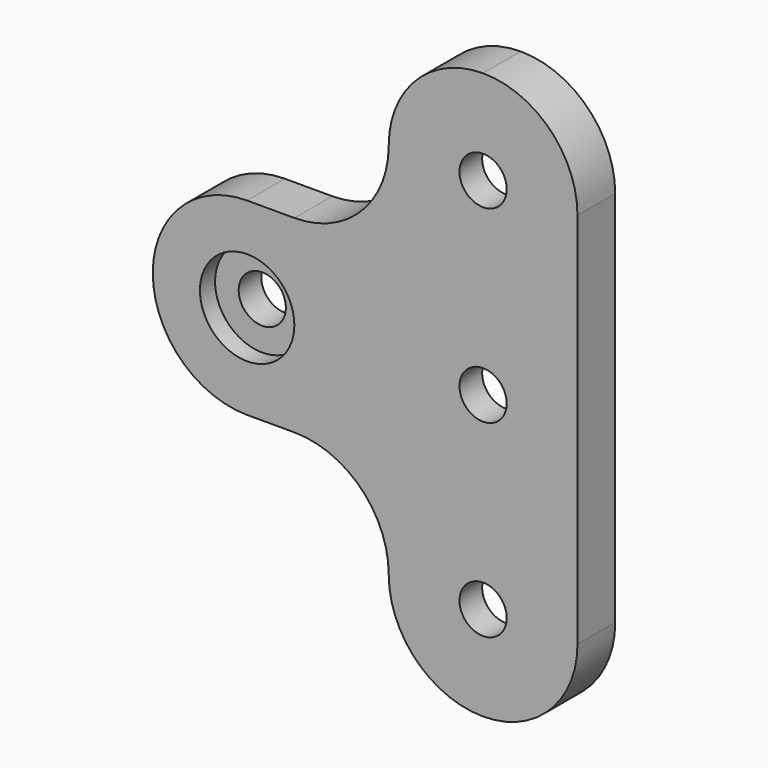
from build123d import *

# Parameters (mm, degrees)
F1_DEPTH       = 5
F2_D           = 5
F2_CBORE_D     = 10
F2_CBORE_DEPTH = 2
F3_R           = 9.99999
F5_D           = 5
F5_CBORE_D     = 10
F5_CBORE_DEPTH = 2


# Not quite as in the source:
# - a fillet or chamfer is up to 0.001 mm smaller than in the source, because OpenCascade refuses the exact size


with BuildPart() as f1:
    # F0 (on Front) → F1 (new body)
    with BuildSketch(Plane.XZ):
        Polygon((15, 10), (-10, 10), (-10, -10), (15, -10), (15, -30), (35, -30), (35, -10), (35, 10), (35, 30), (15, 30), align=None)
    extrude(amount=F1_DEPTH)

    # F2 (through all)
    with Locations(Plane(origin=(0, 0, 0), x_dir=(1, 0, 0), z_dir=(0, 1, 0))):
        with Locations((25, -20), (25, 20), (25, 0)):
            CounterBoreHole(F2_D / 2, F2_CBORE_D / 2, F2_CBORE_DEPTH)

    # F3 (radius 10 in the source; OpenCascade refuses exactly that, so slightly less here)
    f3_edges = [f1.edges().sort_by_distance(p)[0] for p in [
        (35, -2.5, 30),
        (35, -2.5, -30),
        (15, -2.5, -30),
        (15, -2.5, 30),
        (-10, -2.5, 10),
        (-10, -2.5, -10),
        (15, -2.5, 10),
        (15, -2.5, -10),
    ]]
    fillet(f3_edges, radius=F3_R)

    # F5 (through all)
    with Locations(Plane.XZ.offset(5)):
        with Locations((0, 0)):
            CounterBoreHole(F5_D / 2, F5_CBORE_D / 2, F5_CBORE_DEPTH)


solid = f1.part
